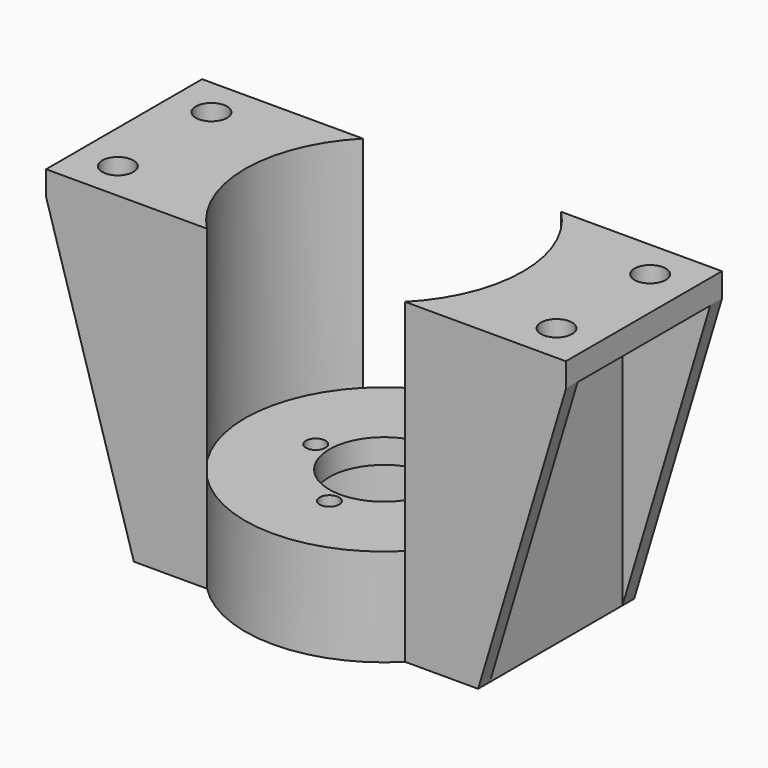
from build123d import *

# Parameters (mm, degrees)
F0_R         = 28.5
F0_R_2       = 18.5
F1_DEPTH     = 15
F2_R         = 28.5
F2_R_2       = 18.5
F3_DEPTH     = 5
F4_R         = 2
F4_R_2       = 11.2
F5_DEPTH     = 25
F7_DEPTH     = 65
F8_W         = 40
F8_H         = 5
F9_DEPTH     = 18
F10_R        = 3.2
F11_DEPTH    = 25
F12_W        = 18
F12_H        = 3
F13_DEPTH    = 60
F14_C1_SIZE2 = 60
F14_C1_SIZE  = 18
F14_C2_SIZE2 = 60
F14_C2_SIZE  = 18
F14_C3_SIZE2 = 60
F14_C3_SIZE  = 18
F14_C4_SIZE2 = 60
F14_C4_SIZE  = 18


# Not quite as in the source:
# - a pattern or mirror of a feature is missing from the dataset's text; its kind, count and spacing are read off the source's solid
# - a feature names something its author has since deleted; it is built from what else it names


with BuildPart() as f1:
    # F0 (on Top) → F1 (new body)
    with BuildSketch(Plane.XY):
        Circle(F0_R)
        Circle(F0_R_2, mode=Mode.SUBTRACT)
    extrude(amount=-F1_DEPTH)

    # F2 (on face) → F3 (join)
    with BuildSketch(Plane.XY):
        Circle(F2_R)
        Circle(F2_R_2, mode=Mode.SUBTRACT)
        Circle(F2_R_2)
    extrude(amount=F3_DEPTH)

    # F4 (on face) → F5 (cut)
    with BuildSketch(Plane.XY.offset(5)):
        with Locations((0, 14)):
            Circle(F4_R)
        Circle(F4_R_2)
        with Locations((-14, 0)):
            Circle(F4_R)
        with Locations((0, -14)):
            Circle(F4_R)
        with Locations((14, 0)):
            Circle(F4_R)
    extrude(amount=-F5_DEPTH, mode=Mode.SUBTRACT)

    # F6 (on face) → F7 (join)
    with BuildSketch(Plane(origin=(0, 0, -15), x_dir=(1, 0, 0), z_dir=(0, 0, -1))):
        with BuildLine():
            ThreePointArc((-20.3039405042, -20), (-28.5, 0), (-20.3039405042, 20))
            Line((-20.3039405042, 20), (-35.3039405042, 20))
            Line((-35.3039405042, 20), (-35.3039405042, -20))
            Line((-35.3039405042, -20), (-20.3039405042, -20))
        make_face()
        with BuildLine():
            Line((35.3039405042, 20), (20.3039405042, 20))
            ThreePointArc((20.3039405042, 20), (26.3715026532, 10.8071202369), (28.5, 0))
            ThreePointArc((28.5, 0), (26.3715026532, -10.8071202369), (20.3039405042, -20))
            Line((20.3039405042, -20), (35.3039405042, -20))
            Line((35.3039405042, -20), (35.3039405042, 20))
        make_face()
    extrude(amount=-F7_DEPTH)

    # F8 (on face) → F9 (join)
    with BuildSketch(Plane.YZ.offset(35.3039405042)):
        with Locations((0, 47.5)):
            Rectangle(F8_W, F8_H)
    f9 = extrude(amount=F9_DEPTH)

    # F9_copies: F9 across plane
    add(f9.mirror(Plane(origin=(0, 0, 0), x_dir=(0, 0, -1), z_dir=(-1, 0, 0))))

    # F10 (on face) → F11 (cut)
    with BuildSketch(Plane(origin=(0, 0, 45), x_dir=(1, 0, 0), z_dir=(0, 0, -1))):
        with Locations((44.9877695576, 12)):
            Circle(F10_R)
        with Locations((44.9877695576, -12)):
            Circle(F10_R)
    f11 = extrude(amount=-F11_DEPTH, mode=Mode.SUBTRACT)

    # F11_copies: F11 across plane
    add(f11.mirror(Plane(origin=(0, 0, 0), x_dir=(0, 0, -1), z_dir=(-1, 0, 0))), mode=Mode.SUBTRACT)

    # F12 (on face) → F13 (join)
    with BuildSketch(Plane(origin=(0, 0, 45), x_dir=(1, 0, 0), z_dir=(0, 0, -1))):
        with Locations((44.3039405042, 18.5)):
            Rectangle(F12_W, F12_H)
        with Locations((44.3039405042, -18.5)):
            Rectangle(F12_W, F12_H)
    f13 = extrude(amount=F13_DEPTH)

    # F13_copies: F13 across plane
    add(f13.mirror(Plane(origin=(0, 0, 0), x_dir=(0, 0, -1), z_dir=(-1, 0, 0))))

    # F14: chamfer of 60 x 18 on 4 edges, made by hand

    # F14_c1
    f14_c1_edges = [f1.edges().sort_by_distance(p)[0] for p in [
        (-53.3039405042, 18.5, -15),
    ]]
    f14_c1_side = f1.faces().sort_by_distance((-52.9439405042, 18.5, -15))[0]
    chamfer(f14_c1_edges, length=F14_C1_SIZE, length2=F14_C1_SIZE2, reference=f14_c1_side)

    # F14_c2
    f14_c2_edges = [f1.edges().sort_by_distance(p)[0] for p in [
        (-53.3039405042, -18.5, -15),
    ]]
    f14_c2_side = f1.faces().sort_by_distance((-52.9439405042, -18.5, -15))[0]
    chamfer(f14_c2_edges, length=F14_C2_SIZE, length2=F14_C2_SIZE2, reference=f14_c2_side)

    # F14_c3
    f14_c3_edges = [f1.edges().sort_by_distance(p)[0] for p in [
        (53.3039405042, -18.5, -15),
    ]]
    f14_c3_side = f1.faces().sort_by_distance((52.9439405042, -18.5, -15))[0]
    chamfer(f14_c3_edges, length=F14_C3_SIZE, length2=F14_C3_SIZE2, reference=f14_c3_side)

    # F14_c4
    f14_c4_edges = [f1.edges().sort_by_distance(p)[0] for p in [
        (53.3039405042, 18.5, -15),
    ]]
    f14_c4_side = f1.faces().sort_by_distance((52.9439405042, 18.5, -15))[0]
    chamfer(f14_c4_edges, length=F14_C4_SIZE, length2=F14_C4_SIZE2, reference=f14_c4_side)


solid = f1.part
